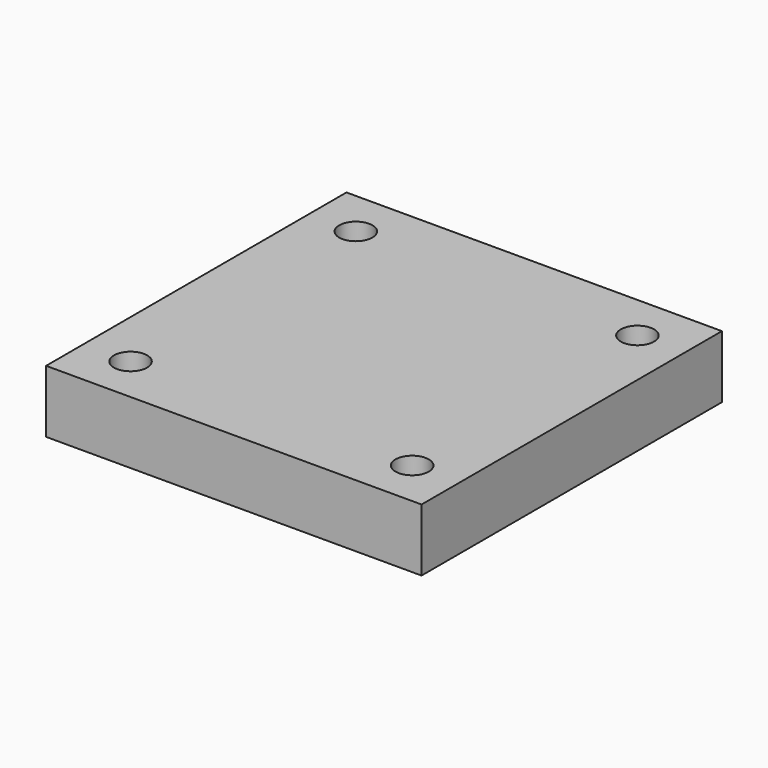
from build123d import *

# Parameters (mm, degrees)
F0_W     = 152.4
F0_H     = 152.4
F1_DEPTH = 25.4
F3_D     = 13.49248


with BuildPart() as f1:
    # F0 (on Top) → F1 (new body)
    with BuildSketch(Plane.XY):
        Rectangle(F0_W, F0_H)
    extrude(amount=-F1_DEPTH)

    # F3 (through all)
    with Locations(Plane.XY):
        with Locations((-57.15, 57.15), (57.15, 57.15), (-57.15, -57.15), (57.15, -57.15)):
            Hole(F3_D / 2)


solid = f1.part
